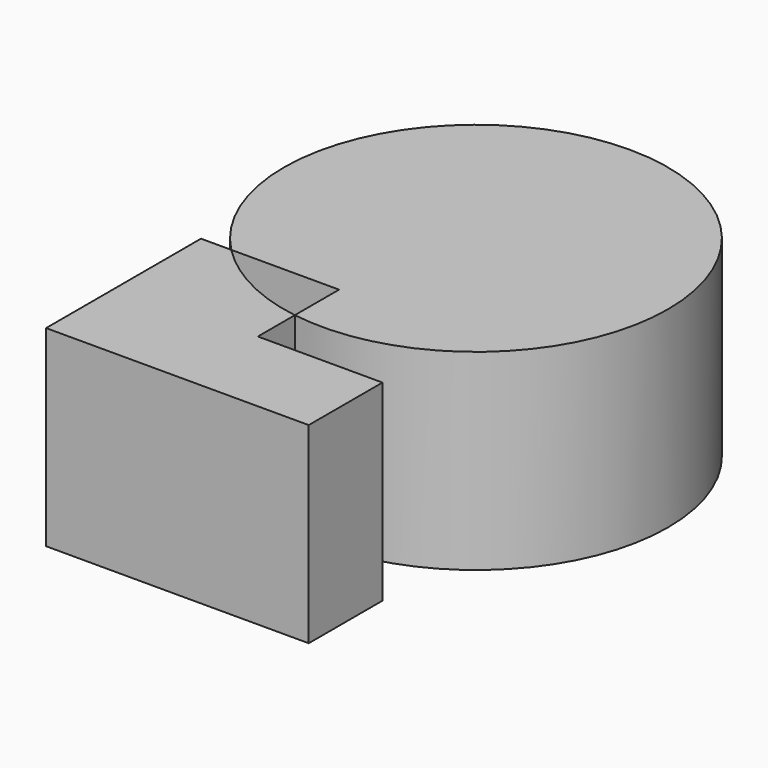
from build123d import *

# Parameters (mm, degrees)
F2_DEPTH = 30


with BuildPart() as f2:
    # F1 (on face) → F2 (new body, symmetric)
    with BuildSketch(Plane.XY):
        with BuildLine():
            ThreePointArc((43.1228913367, 43.2291245988), (91.3251453141, 56.9848894443), (112.2641316056, 102.5286838412))
            ThreePointArc((112.2641316056, 102.5286838412), (94.6905384768, 144.9550907124), (52.2641316056, 162.5286838412))
            ThreePointArc((52.2641316056, 162.5286838412), (-3.0640101085, 125.7406793276), (9.4549124143, 60.4885749899))
            Line((9.4549124143, 60.4885749899), (43.1228913367, 60.4885749899))
            Line((43.1228913367, 60.4885749899), (43.1228913367, 43.2291245988))
        make_face()
    extrude(amount=F2_DEPTH, both=True)


with BuildPart() as f2b:
    # F1 (on face) → F2, piece 2 (new body, symmetric)
    with BuildSketch(Plane.XY):
        with BuildLine():
            Line((43.1228913367, 28.7836860266), (43.1228913367, 43.2291245988))
            ThreePointArc((43.1228913367, 43.2291245988), (24.8928927501, 49.1356572973), (9.4549124143, 60.4885749899))
            Line((9.4549124143, 60.4885749899), (0, 60.4885749899))
            Line((0, 60.4885749899), (0, 0))
            Line((0, 0), (82.0480691682, 0))
            Line((82.0480691682, 0), (82.0480691682, 28.7836860266))
            Line((82.0480691682, 28.7836860266), (43.1228913367, 28.7836860266))
        make_face()
    extrude(amount=F2_DEPTH, both=True)


solid = Compound([f2.part, f2b.part])
